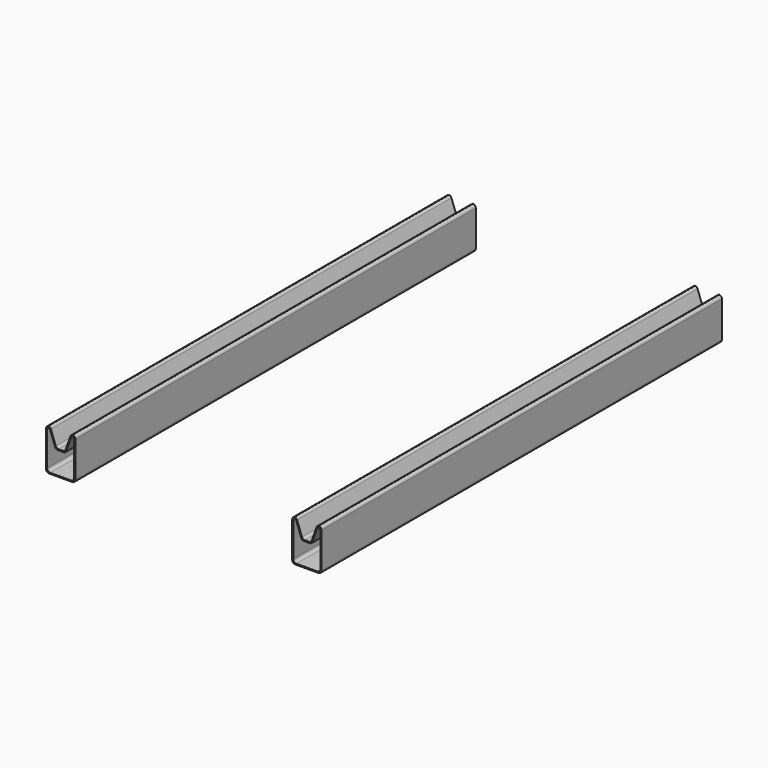
from build123d import *

# Parameters (mm, degrees)
F1_DEPTH    = 6000
F2_T        = -26
F2_2_T      = -26
F3_T1_DEPTH = 12000
F3_T3_DEPTH = 12350
F3_T5_DEPTH = 12245.0726383734
F4_T1_DEPTH = 12000
F4_T3_DEPTH = 12350
F4_T5_DEPTH = 12245.0726383734


# Not quite as in the source:
# - a fillet or chamfer that OpenCascade refuses, or shapes differently, is made with other operations: its cross-section is extruded or revolved along the edge and cut away or added
# - a feature names something its author has since deleted; it is built from what else it names


with BuildPart() as f1:
    # F0 (on Front) → F1 (new body, symmetric)
    with BuildSketch(Plane.XZ):
        Polygon((2700, 500), (2600, 500), (2600, 200), (2600, 0), (2600, -200), (2600, -500), (3300, -500), (3300, 500), (3200, 500), (3050, 87.8783870818), (2850, 87.8783870818), align=None)
    extrude(amount=F1_DEPTH, both=True)

    # F2
    f2_openings = [f1.faces().sort_by_distance(p)[0] for p in [
        (2950, -6000, -83.929869),
        (2950, 6000, -83.929869),
    ]]
    offset(amount=F2_T, openings=f2_openings, kind=Kind.INTERSECTION)

    # F3: fillet of radius 70 on 16 edges, made by hand

    # F3_s2 → F3_t1 (join)
    with BuildSketch(Plane.XZ.offset(-6000)):
        with BuildLine():
            ThreePointArc((2833.2360442197, 133.936977049), (2858.8641771301, 100.5377439816), (2899.0145276747, 87.8783870818))
            Line((2899.0145276747, 87.8783870818), (2850, 87.8783870818))
            Line((2850, 87.8783870818), (2833.2360442197, 133.936977049))
        make_face()
        with BuildLine():
            ThreePointArc((2696, -474), (2646.5025253169, -453.4974746831), (2626, -404))
            Line((2626, -404), (2626, -474))
            Line((2626, -474), (2696, -474))
        make_face()
        with BuildLine():
            ThreePointArc((3201.4414402131, 427.9414100328), (3227.0695731236, 461.3406431002), (3267.2199236681, 474))
            Line((3267.2199236681, 474), (3218.2053959935, 474))
            Line((3218.2053959935, 474), (3201.4414402131, 427.9414100328))
        make_face()
        with BuildLine():
            ThreePointArc((3204, 474), (3253.4974746831, 453.4974746831), (3274, 404))
            Line((3274, 404), (3274, 474))
            Line((3274, 474), (3204, 474))
        make_face()
        with BuildLine():
            ThreePointArc((2698.5585597869, 427.9414100328), (2672.9304268764, 461.3406431002), (2632.7800763319, 474))
            Line((2632.7800763319, 474), (2681.7946040065, 474))
            Line((2681.7946040065, 474), (2698.5585597869, 427.9414100328))
        make_face()
        with BuildLine():
            ThreePointArc((2626, 404), (2646.5025253169, 453.4974746831), (2696, 474))
            Line((2696, 474), (2626, 474))
            Line((2626, 474), (2626, 404))
        make_face()
        with BuildLine():
            ThreePointArc((3274, -404), (3253.4974746831, -453.4974746831), (3204, -474))
            Line((3204, -474), (3274, -474))
            Line((3274, -474), (3274, -404))
        make_face()
        with BuildLine():
            ThreePointArc((3000.9854723253, 87.8783870818), (3041.1358228699, 100.5377439816), (3066.7639557803, 133.936977049))
            Line((3066.7639557803, 133.936977049), (3050, 87.8783870818))
            Line((3050, 87.8783870818), (3000.9854723253, 87.8783870818))
        make_face()
    extrude(amount=F3_T1_DEPTH)

    # F3_s4 → F3_t3 (cut)
    with BuildSketch(Plane.XZ.offset(-6175)):
        with BuildLine():
            ThreePointArc((3300, 430), (3279.4974746831, 479.4974746831), (3230, 500))
            Line((3230, 500), (3300, 500))
            Line((3300, 500), (3300, 430))
        make_face()
        with BuildLine():
            ThreePointArc((2670, 500), (2620.5025253169, 479.4974746831), (2600, 430))
            Line((2600, 430), (2600, 500))
            Line((2600, 500), (2670, 500))
        make_face()
        with BuildLine():
            ThreePointArc((3230, -500), (3279.4974746831, -479.4974746831), (3300, -430))
            Line((3300, -430), (3300, -500))
            Line((3300, -500), (3230, -500))
        make_face()
        with BuildLine():
            ThreePointArc((2600, -430), (2620.5025253169, -479.4974746831), (2670, -500))
            Line((2670, -500), (2600, -500))
            Line((2600, -500), (2600, -430))
        make_face()
    extrude(amount=F3_T3_DEPTH, mode=Mode.SUBTRACT)

    # F3_s6 → F3_t5 (cut)
    with BuildSketch(Plane.XZ.offset(-6122.5363191867)):
        with BuildLine():
            ThreePointArc((2716.7639557803, 453.9414100328), (2691.1358228699, 487.3406431002), (2650.9854723253, 500))
            Line((2650.9854723253, 500), (2700, 500))
            Line((2700, 500), (2716.7639557803, 453.9414100328))
        make_face()
        with BuildLine():
            ThreePointArc((3183.2360442197, 453.9414100328), (3208.8641771301, 487.3406431002), (3249.0145276747, 500))
            Line((3249.0145276747, 500), (3200, 500))
            Line((3200, 500), (3183.2360442197, 453.9414100328))
        make_face()
        with BuildLine():
            ThreePointArc((3084.9693517738, 107.936977049), (3059.3412188633, 74.5377439816), (3019.1908683188, 61.8783870818))
            Line((3019.1908683188, 61.8783870818), (3068.2053959935, 61.8783870818))
            Line((3068.2053959935, 61.8783870818), (3084.9693517738, 107.936977049))
        make_face()
        with BuildLine():
            ThreePointArc((2815.0306482262, 107.936977049), (2840.6587811367, 74.5377439816), (2880.8091316812, 61.8783870818))
            Line((2880.8091316812, 61.8783870818), (2831.7946040065, 61.8783870818))
            Line((2831.7946040065, 61.8783870818), (2815.0306482262, 107.936977049))
        make_face()
    extrude(amount=F3_T5_DEPTH, mode=Mode.SUBTRACT)


with BuildPart() as f1b:
    # F0 (on Front) → F1, piece 2 (new body, symmetric)
    with BuildSketch(Plane.XZ):
        Polygon((-2600, -200), (-2600, 0), (-2600, 200), (-2600, 500), (-2700, 500), (-2850, 87.8783870818), (-3050, 87.8783870818), (-3200, 500), (-3300, 500), (-3300, -500), (-2600, -500), align=None)
    extrude(amount=F1_DEPTH, both=True)

    # F2#2
    f2_2_openings = [f1b.faces().sort_by_distance(p)[0] for p in [
        (-2950, -6000, -83.929869),
        (-2950, 6000, -83.929869),
    ]]
    offset(amount=F2_2_T, openings=f2_2_openings, kind=Kind.INTERSECTION)

    # F4: fillet of radius 70 on 16 edges, made by hand

    # F4_s2 → F4_t1 (join)
    with BuildSketch(Plane.XZ.offset(-6000)):
        with BuildLine():
            ThreePointArc((-3066.7639557803, 133.936977049), (-3041.1358228699, 100.5377439816), (-3000.9854723253, 87.8783870818))
            Line((-3000.9854723253, 87.8783870818), (-3050, 87.8783870818))
            Line((-3050, 87.8783870818), (-3066.7639557803, 133.936977049))
        make_face()
        with BuildLine():
            ThreePointArc((-3274, -404), (-3253.4974746831, -453.4974746831), (-3204, -474))
            Line((-3204, -474), (-3274, -474))
            Line((-3274, -474), (-3274, -404))
        make_face()
        with BuildLine():
            ThreePointArc((-2626, -404), (-2646.5025253169, -453.4974746831), (-2696, -474))
            Line((-2696, -474), (-2626, -474))
            Line((-2626, -474), (-2626, -404))
        make_face()
        with BuildLine():
            ThreePointArc((-2899.0145276747, 87.8783870818), (-2858.8641771301, 100.5377439816), (-2833.2360442197, 133.936977049))
            Line((-2833.2360442197, 133.936977049), (-2850, 87.8783870818))
            Line((-2850, 87.8783870818), (-2899.0145276747, 87.8783870818))
        make_face()
        with BuildLine():
            ThreePointArc((-3267.2199236681, 474), (-3227.0695731236, 461.3406431002), (-3201.4414402131, 427.9414100328))
            Line((-3201.4414402131, 427.9414100328), (-3218.2053959935, 474))
            Line((-3218.2053959935, 474), (-3267.2199236681, 474))
        make_face()
        with BuildLine():
            ThreePointArc((-2698.5585597869, 427.9414100328), (-2672.9304268764, 461.3406431002), (-2632.7800763319, 474))
            Line((-2632.7800763319, 474), (-2681.7946040065, 474))
            Line((-2681.7946040065, 474), (-2698.5585597869, 427.9414100328))
        make_face()
        with BuildLine():
            ThreePointArc((-2626, 404), (-2646.5025253169, 453.4974746831), (-2696, 474))
            Line((-2696, 474), (-2626, 474))
            Line((-2626, 474), (-2626, 404))
        make_face()
        with BuildLine():
            ThreePointArc((-3274, 404), (-3253.4974746831, 453.4974746831), (-3204, 474))
            Line((-3204, 474), (-3274, 474))
            Line((-3274, 474), (-3274, 404))
        make_face()
    extrude(amount=F4_T1_DEPTH)

    # F4_s4 → F4_t3 (cut)
    with BuildSketch(Plane.XZ.offset(-6175)):
        with BuildLine():
            ThreePointArc((-2600, 430), (-2620.5025253169, 479.4974746831), (-2670, 500))
            Line((-2670, 500), (-2600, 500))
            Line((-2600, 500), (-2600, 430))
        make_face()
        with BuildLine():
            ThreePointArc((-3300, 430), (-3279.4974746831, 479.4974746831), (-3230, 500))
            Line((-3230, 500), (-3300, 500))
            Line((-3300, 500), (-3300, 430))
        make_face()
        with BuildLine():
            ThreePointArc((-2600, -430), (-2620.5025253169, -479.4974746831), (-2670, -500))
            Line((-2670, -500), (-2600, -500))
            Line((-2600, -500), (-2600, -430))
        make_face()
        with BuildLine():
            ThreePointArc((-3230, -500), (-3279.4974746831, -479.4974746831), (-3300, -430))
            Line((-3300, -430), (-3300, -500))
            Line((-3300, -500), (-3230, -500))
        make_face()
    extrude(amount=F4_T3_DEPTH, mode=Mode.SUBTRACT)

    # F4_s6 → F4_t5 (cut)
    with BuildSketch(Plane.XZ.offset(-6122.5363191867)):
        with BuildLine():
            ThreePointArc((-2650.9854723253, 500), (-2691.1358228699, 487.3406431002), (-2716.7639557803, 453.9414100328))
            Line((-2716.7639557803, 453.9414100328), (-2700, 500))
            Line((-2700, 500), (-2650.9854723253, 500))
        make_face()
        with BuildLine():
            ThreePointArc((-3249.0145276747, 500), (-3208.8641771301, 487.3406431002), (-3183.2360442197, 453.9414100328))
            Line((-3183.2360442197, 453.9414100328), (-3200, 500))
            Line((-3200, 500), (-3249.0145276747, 500))
        make_face()
        with BuildLine():
            ThreePointArc((-2815.0306482262, 107.936977049), (-2840.6587811367, 74.5377439816), (-2880.8091316812, 61.8783870818))
            Line((-2880.8091316812, 61.8783870818), (-2831.7946040065, 61.8783870818))
            Line((-2831.7946040065, 61.8783870818), (-2815.0306482262, 107.936977049))
        make_face()
        with BuildLine():
            ThreePointArc((-3019.1908683188, 61.8783870818), (-3059.3412188633, 74.5377439816), (-3084.9693517738, 107.936977049))
            Line((-3084.9693517738, 107.936977049), (-3068.2053959935, 61.8783870818))
            Line((-3068.2053959935, 61.8783870818), (-3019.1908683188, 61.8783870818))
        make_face()
    extrude(amount=F4_T5_DEPTH, mode=Mode.SUBTRACT)


solid = Compound([f1.part, f1b.part])
